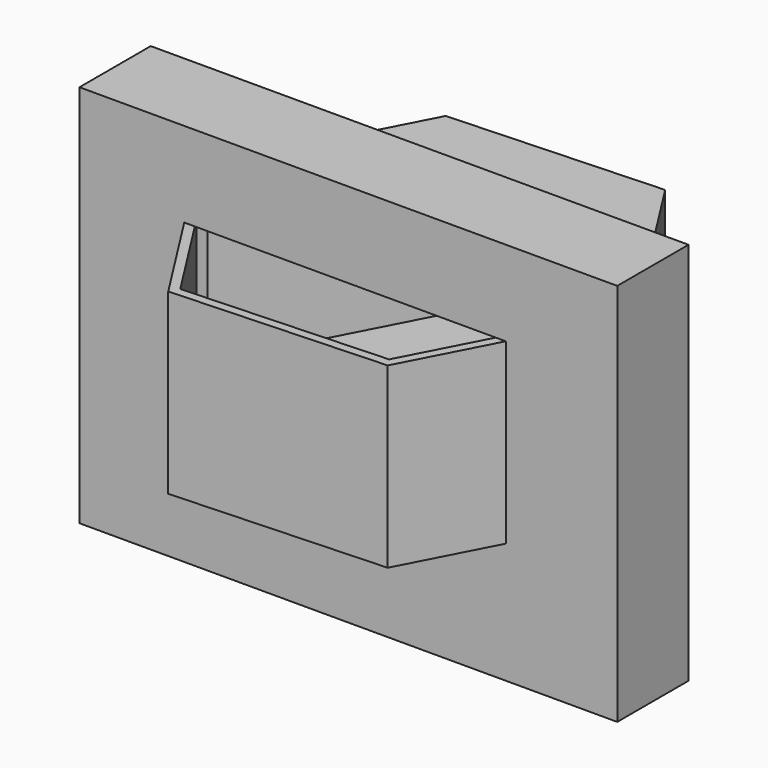
from build123d import *

# Parameters (mm, degrees)
F1_DEPTH = 50.8
F2_W     = 153.3701941371
F2_H     = 109.4799749553
F3_DEPTH = 25.4
F4_T     = -2.54


# Not quite as in the source:
# - a shell that OpenCascade refuses in one call is made with other operations: the cavity is built on its own and cut out


with BuildPart() as f1:
    # F0 (on Top) → F1 (new body)
    with BuildSketch(Plane.XY):
        Polygon((32.5404184413, -50.9185224387), (60.4496595907, 2.769324145), (27.9092411494, 53.7833592726), (-32.5404184413, 51.1095478164), (-60.4496595907, -2.5782987673), (-27.9092411494, -53.5923338949), align=None)
    extrude(amount=F1_DEPTH)

    # F2 (on Front) → F3 (join)
    with BuildSketch(Plane.XZ):
        with Locations((0.9111128747, 20.3165654093)):
            Rectangle(F2_W, F2_H)
    extrude(amount=F3_DEPTH)

    # F4: a shell. OpenCascade refuses it in one call, so the cavity is built on its own and cut out:
    # the body offset inwards by the wall thickness, plus a prism from it out through each open face.
    f4_core = offset(f1.part, amount=F4_T, kind=Kind.INTERSECTION, mode=Mode.PRIVATE)
    f4_exits = [f4_core.faces().sort_by_distance(p)[0] for p in [
        (0.261081, -35.353201, 48.26),
    ]]
    add(f4_core, mode=Mode.SUBTRACT)
    extrude(f4_exits, amount=-F4_T, mode=Mode.SUBTRACT)


solid = f1.part
